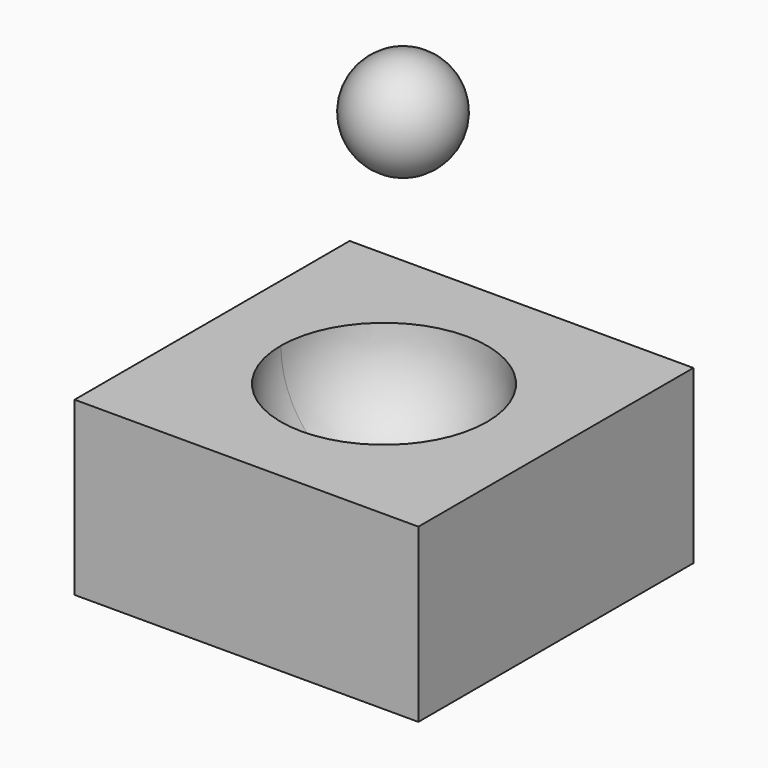
from build123d import *
from build123d import SkipClean  # not in build123d's __all__

# Parameters (mm, degrees)
F0_W     = 100
F0_H     = 100
F1_DEPTH = 50


with BuildPart() as f1:
    # F0 (on Top) → F1 (new body)
    with BuildSketch(Plane.XY):
        with Locations((-50, 0)):
            Rectangle(F0_W, F0_H)
    extrude(amount=F1_DEPTH)

    # F2 (on Front) → F3 (revolve, cut)
    with BuildSketch(Plane.XZ):
        with BuildLine():
            Line((-20, 50), (-80, 50))
            ThreePointArc((-80, 50), (-50, 20), (-20, 50))
        make_face()
    with SkipClean():  # cleaning this boolean's faces spoils the solid; the shape is the same uncleaned
        revolve(axis=Axis((-50, 0, 50), (1, 0, 0)), mode=Mode.SUBTRACT)


with BuildPart() as f6:
    # F5 (on Front) → F6 (revolve)
    with BuildSketch(Plane.XZ):
        with BuildLine():
            Line((-44.4710201616, 106.3925326908), (-44.4710201616, 136.3925326908))
            ThreePointArc((-44.4710201616, 136.3925326908), (-59.4710201616, 121.3925326908), (-44.4710201616, 106.3925326908))
        make_face()
    revolve(axis=Axis((-44.4710201616, 0, 121.3925326908), (0, 0, -1)))


solid = Compound([f1.part, f6.part])
